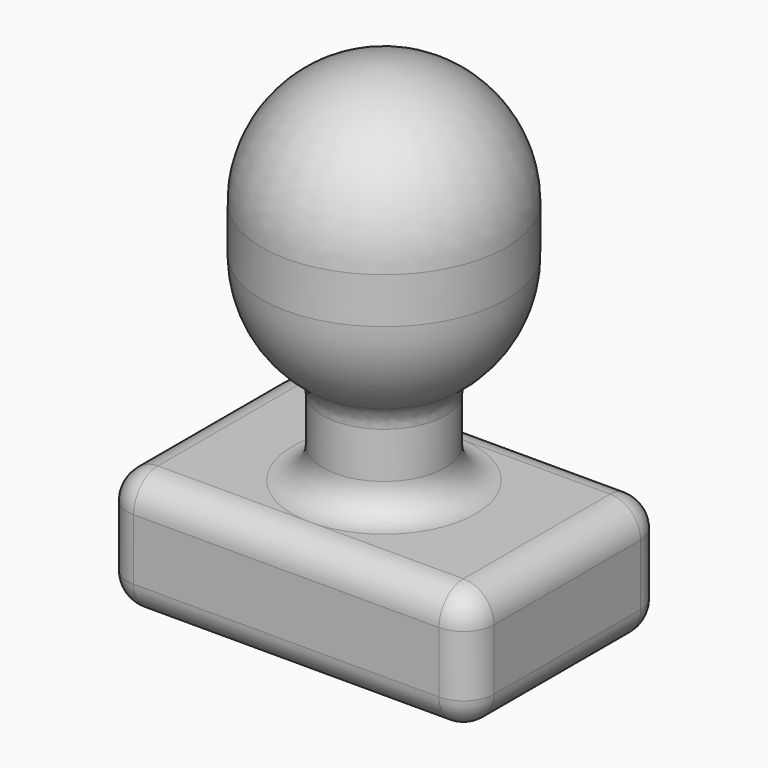
from build123d import *

# Parameters (mm, degrees)
F0_W     = 152.4
F0_H     = 101.6
F1_DEPTH = 50.8
F2_W     = 50.7960162224
F2_H     = 19.05
F4_R     = 12.69999


# Not quite as in the source:
# - a fillet or chamfer is up to 0.001 mm smaller than in the source, because OpenCascade refuses the exact size
# - a feature names something its author has since deleted; it is built from what else it names


with BuildPart() as f1:
    # F0 (on Top) → F1 (new body)
    with BuildSketch(Plane.XY):
        Rectangle(F0_W, F0_H)
    extrude(amount=-F1_DEPTH)

    # F2 (on Front) → F3 (revolve)
    with BuildSketch(Plane.XZ):
        with BuildLine():
            Line((0, 31.7539837776), (0, 0))
            Line((0, 0), (25.4, 0))
            Line((25.4, 0), (25.4, 38.560509618))
            ThreePointArc((25.4, 38.560509618), (13.1480872565, 33.4851137211), (0, 31.7539837776))
        make_face()
        with BuildLine():
            Line((0, 82.55), (0, 31.7539837776))
            ThreePointArc((0, 31.7539837776), (13.1480872565, 33.4851137211), (25.4, 38.560509618))
            ThreePointArc((25.4, 38.560509618), (43.9912154647, 57.1529878527), (50.7960162224, 82.55))
            Line((50.7960162224, 82.55), (0, 82.55))
        make_face()
        with Locations((25.3980081112, 92.075)):
            Rectangle(F2_W, F2_H)
        with BuildLine():
            Line((0, 152.3999998438), (0, 101.6))
            Line((0, 101.6), (50.7960162224, 101.6))
            ThreePointArc((50.7960162224, 101.6), (35.9184491572, 137.5196159786), (0, 152.3999998438))
        make_face()
    revolve(axis=Axis((0, 0, 76.1999999219), (0, 0, 1)))

    # F4 (radius 12.7 in the source; OpenCascade refuses exactly that, so slightly less here)
    f4_edges = [f1.edges().sort_by_distance(p)[0] for p in [
        (0, 50.8, 0),
        (76.2, 0, 0),
        (-76.2, 0, 0),
        (0, -50.8, 0),
        (-25.4, 0, 0),
        (-76.2, -50.8, -25.4),
        (76.2, -50.8, -25.4),
        (0, -50.8, -50.8),
        (-76.2, 50.8, -25.4),
        (-76.2, 0, -50.8),
        (76.2, 50.8, -25.4),
        (0, 50.8, -50.8),
        (76.2, 0, -50.8),
        (-25.4, 0, 38.56051),
        (25.4, 0, 19.280255),
    ]]
    fillet(f4_edges, radius=F4_R)


solid = f1.part
